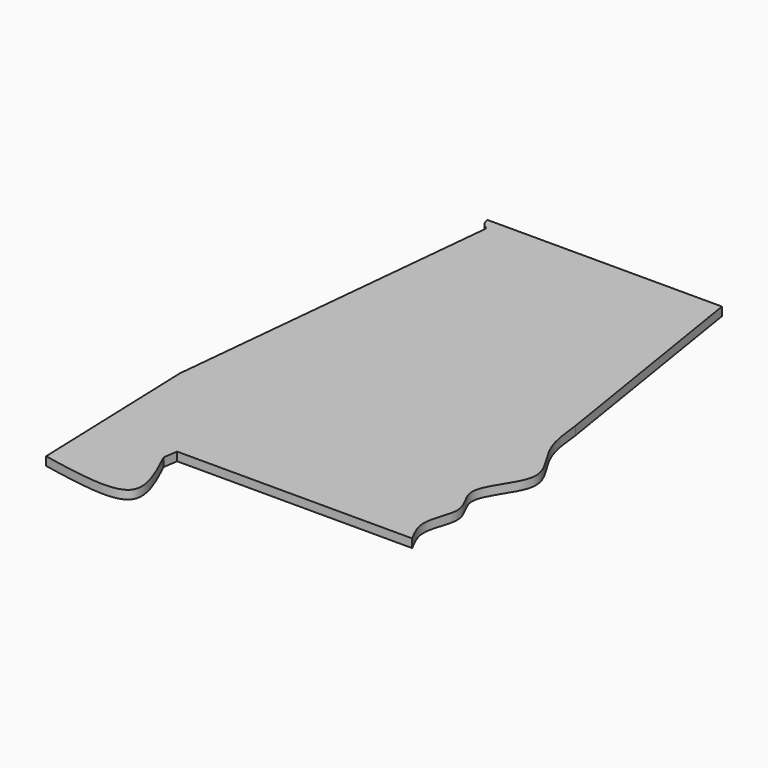
from build123d import *

# Parameters (mm, degrees)
F1_DEPTH = 2


# Not quite as in the source:
# - a feature of the source that left no trace in its solid (it failed there, or was rolled back) is left out


with BuildPart() as f1:
    # F0 (on Top) → F1 (new body)
    with BuildSketch(Plane.XY):
        with BuildLine():
            add(Edge.make_bspline(
                [(-32.4043067872, 59.2193437133), (-32.9455181975, 59.581828676), (-33.9978316805, 60.2866323929), (-34.2577204684, 61.4241960814), (-34.3839468261, 61.9767036454)],
                knots=[0, 0, 0, 0, 0.5143062586, 1, 1, 1, 1], degree=3))
            Line((-32.4043067872, 59.2193437133), (-40.29759312, -20.3441163994))
            Line((-40.29759312, -20.3441163994), (-38.8994998628, -61.1876496762))
            add(Edge.make_bspline(
                [(-21.8826408634, -48.1355482657), (-19.2255669001, -53.7660393666), (-13.3709239797, -66.1723612522), (-29.8818826365, -62.948430269), (-38.8994998628, -61.1876496762)],
                knots=[0, 0, 0, 0, 0.4538404817, 1, 1, 1, 1], degree=3))
            Line((-21.8826408634, -48.1355482657), (-21.3790618005, -44.8284622711))
            Line((-21.3790618005, -44.8284622711), (33.52433514, -44.8284622711))
            add(Edge.make_bspline(
                [(28.984086711, 8.4774404124), (29.3516469163, 4.8591304728), (30.0850907545, -2.3609850111), (39.1649832019, -11.8903794357), (27.4292491551, -23.0695594567), (34.9658128507, -30.0388830909), (29.9798094231, -38.3642272099), (32.3760551751, -42.734317045), (33.52433514, -44.8284622711)],
                knots=[0, 0, 0, 0, 0.1802729556, 0.3597236224, 0.5505400077, 0.7005520483, 0.8565046665, 1, 1, 1, 1], degree=3))
            Line((28.984086711, 8.4774404124), (20.4112881077, 61.9767036454))
            Line((20.4112881077, 61.9767036454), (-34.3839468261, 61.9767036454))
        make_face()
    extrude(amount=F1_DEPTH)


solid = f1.part
